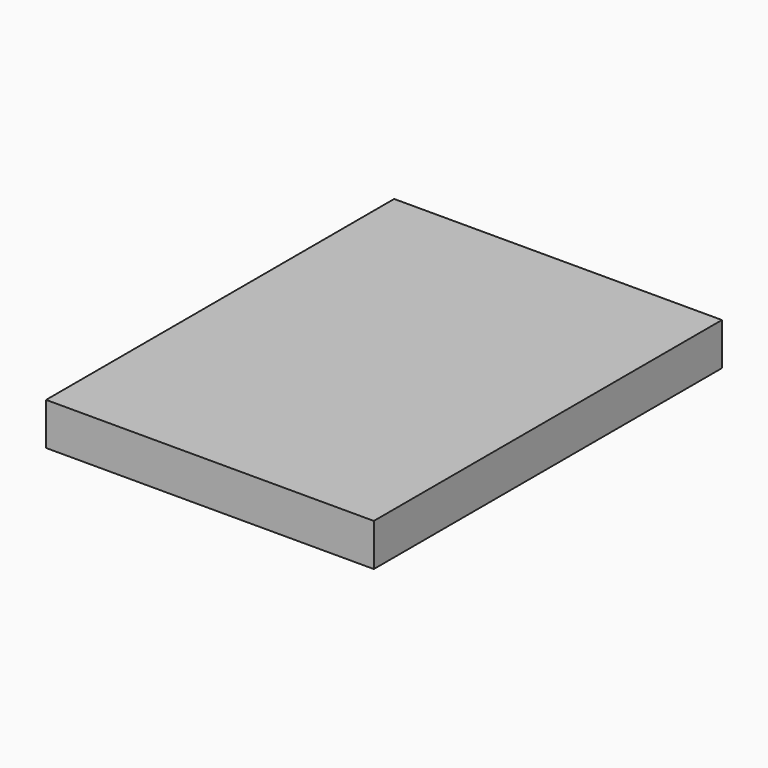
from build123d import *

# Parameters (mm, degrees)
F0_W     = 73.66
F0_H     = 97.79
F1_DEPTH = 9.525


# Not quite as in the source:
# - a length typed as a fraction of an inch, garbled in the dataset ("3 / 203.2 mm" for 3/8 in), is restored


with BuildPart() as f1:
    # F0 (on Top) → F1 (new body)
    with BuildSketch(Plane.XY):
        Rectangle(F0_W, F0_H)
    extrude(amount=F1_DEPTH)

    # F2 (on Right) → F3 (revolve)
    with BuildSketch(Plane.YZ):
        Polygon((35.179, 0), (33.401, 0), (33.401, -5.334), (37.5285, -5.334), (37.5285, -1.524), (35.179, -1.524), align=None)
    revolve(axis=Axis((0, 33.401, -2.667), (0, 0, -1)))

    # F2 (on Right) → F4 (revolve)
    with BuildSketch(Plane.YZ):
        Polygon((-33.401, 0), (-35.179, 0), (-35.179, -1.524), (-37.5285, -1.524), (-37.5285, -5.334), (-33.401, -5.334), align=None)
    revolve(axis=Axis((0, -33.401, -2.667), (0, 0, -1)))


solid = f1.part
